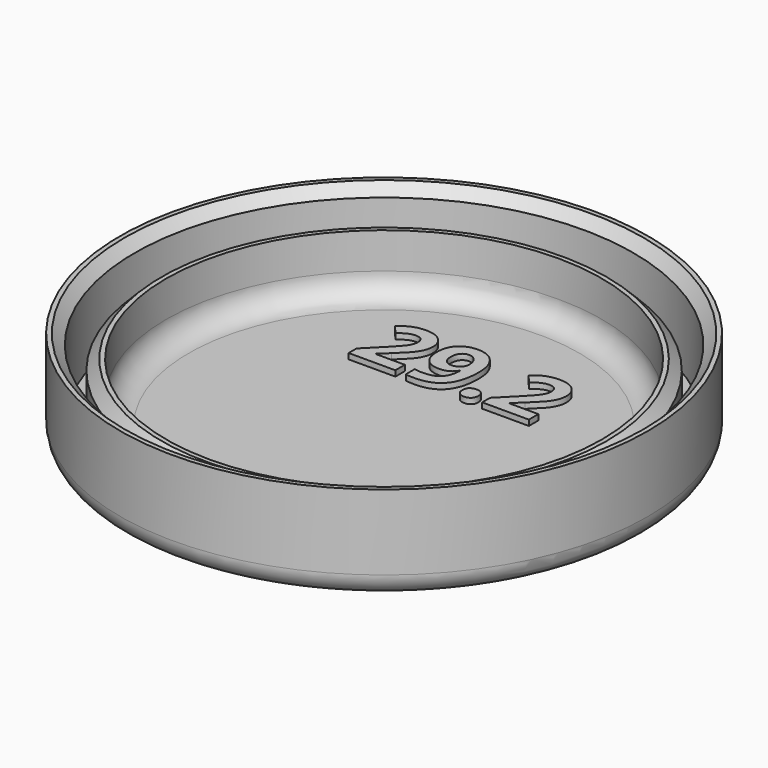
from build123d import *

# Parameters (mm, degrees)
F2_TEXT_SIZE = 8.3333333333
F3_DEPTH     = 0.5


# Not quite as in the source:
# - Text() gives the source's letters only with a copy of the font that has no kerning and outlines rounded to 1/6400 em; it was checked with that copy


with BuildPart() as f1:
    # F0 (on Front) → F1 (revolve)
    with BuildSketch(Plane.XZ):
        with BuildLine():
            Line((0, 1.5), (0, 0))
            Line((0, 0), (21.5, 0))
            ThreePointArc((21.5, 0), (22.9142135624, 0.5857864376), (23.5, 2))
            Line((23.5, 2), (23.5, 8.7))
            Line((23.5, 8.7), (23.1, 8.7))
            Line((23.1, 8.7), (22.2, 7.8))
            Line((22.2, 7.8), (22.2, 1.5))
            Line((22.2, 1.5), (20.7, 1.5))
            Line((20.7, 1.5), (20.7, 5.8))
            Line((20.7, 5.8), (19.8, 6.7))
            Line((19.8, 6.7), (19.4, 6.7))
            Line((19.4, 6.7), (19.4, 3.5))
            ThreePointArc((19.4, 3.5), (18.8142135624, 2.0857864376), (17.4, 1.5))
            Line((17.4, 1.5), (0, 1.5))
        make_face()
    revolve(axis=Axis((0, 0, 0.75), (0, 0, 1)))

    # F2 (on face) → F3 (join)
    with BuildSketch(Plane.XY.offset(1.5)):
        with Locations((-8.4609375, 6.2138572465)):
            Text('29.2', F2_TEXT_SIZE, font='Open Sans', font_style=FontStyle.BOLD, text_align=(TextAlign.LEFT, TextAlign.BOTTOM))
    extrude(amount=F3_DEPTH)


solid = f1.part
